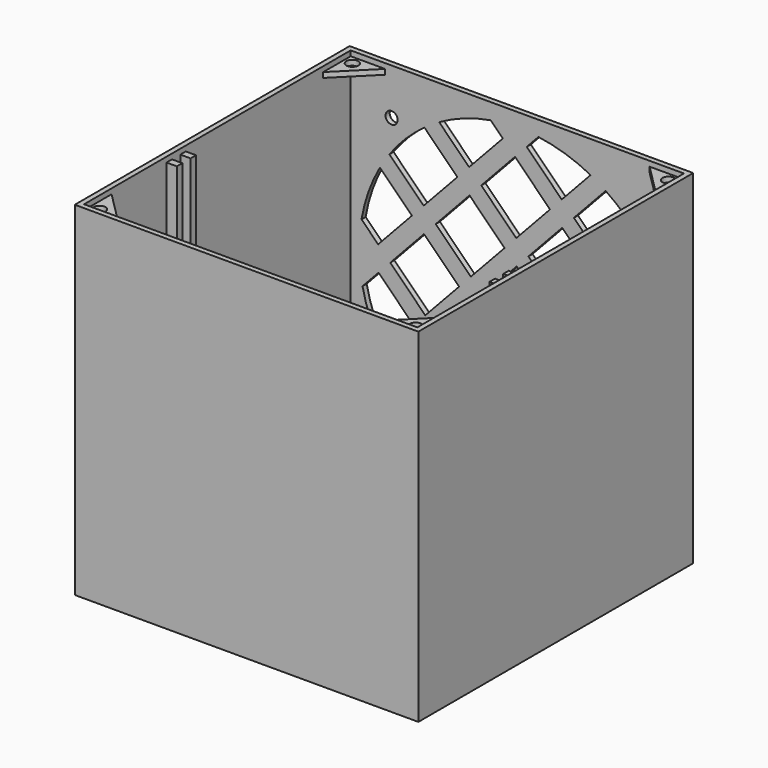
from build123d import *

# Parameters (mm, degrees)
F0_W      = 100
F0_H      = 100
F0_R      = 5
F0_W_2    = 3
F0_H_2    = 2
F1_DEPTH  = 1.5
F2_W      = 100
F2_H      = 100
F3_DEPTH  = 98.5
F2_W_2    = 3
F2_H_2    = 2
F4_DEPTH  = 97
F5_R      = 1.75
F6_DEPTH  = 1.5
F7_R      = 1.75
F8_DEPTH  = 3
F8_FACE_R = 1.75
F9_DEPTH  = 1.5
F2_R      = 3.5
F2_R_2    = 1.75
F10_DEPTH = 7


with BuildPart() as f1:
    # F0 (on Top) → F1 (new body)
    with BuildSketch(Plane.XY):
        with Locations((50, 50)):
            Rectangle(F0_W, F0_H)
        Polygon((98.5, 1.5), (1.5, 1.5), (1.5, 31.5), (1.5, 33.5), (1.5, 36.5), (1.5, 38.5), (1.5, 98.5), (98.5, 98.5), (98.5, 38.5), (98.5, 36.5), (98.5, 33.5), (98.5, 31.5), align=None, mode=Mode.SUBTRACT)
        Polygon((1.5, 31.5), (1.5, 1.5), (98.5, 1.5), (98.5, 31.5), (95.5, 31.5), (95.5, 33.5), (98.5, 33.5), (98.5, 36.5), (95.5, 36.5), (95.5, 38.5), (98.5, 38.5), (98.5, 98.5), (1.5, 98.5), (1.5, 38.5), (4.5, 38.5), (4.5, 36.5), (1.5, 36.5), (1.5, 33.5), (4.5, 33.5), (4.5, 31.5), align=None)
        with Locations((20.9, 53.5)):
            Circle(F0_R, mode=Mode.SUBTRACT)
        with Locations((40.3, 53.5)):
            Circle(F0_R, mode=Mode.SUBTRACT)
        with Locations((20.9, 78.5)):
            Circle(F0_R, mode=Mode.SUBTRACT)
        with Locations((59.7, 53.5)):
            Circle(F0_R, mode=Mode.SUBTRACT)
        with Locations((79.1, 53.5)):
            Circle(F0_R, mode=Mode.SUBTRACT)
        with Locations((79.1, 78.5)):
            Circle(F0_R, mode=Mode.SUBTRACT)
        with Locations((3, 37.5)):
            Rectangle(F0_W_2, F0_H_2)
        with Locations((3, 32.5)):
            Rectangle(F0_W_2, F0_H_2)
        with Locations((97, 37.5)):
            Rectangle(F0_W_2, F0_H_2)
        with Locations((97, 32.5)):
            Rectangle(F0_W_2, F0_H_2)
    extrude(amount=F1_DEPTH)

    # F2 (on face) → F3 (join)
    with BuildSketch(Plane.XY.offset(1.5)):
        with Locations((50, 50)):
            Rectangle(F2_W, F2_H)
        Polygon((98.5, 1.5), (1.5, 1.5), (1.5, 31.5), (1.5, 33.5), (1.5, 36.5), (1.5, 38.5), (1.5, 98.5), (98.5, 98.5), (98.5, 38.5), (98.5, 36.5), (98.5, 33.5), (98.5, 31.5), align=None, mode=Mode.SUBTRACT)
    extrude(amount=F3_DEPTH)

    # F2 (on face) → F4 (join)
    with BuildSketch(Plane.XY.offset(1.5)):
        with Locations((50, 50)):
            Rectangle(F2_W, F2_H)
        Polygon((98.5, 1.5), (1.5, 1.5), (1.5, 31.5), (1.5, 33.5), (1.5, 36.5), (1.5, 38.5), (1.5, 98.5), (98.5, 98.5), (98.5, 38.5), (98.5, 36.5), (98.5, 33.5), (98.5, 31.5), align=None, mode=Mode.SUBTRACT)
        with Locations((3, 37.5)):
            Rectangle(F2_W_2, F2_H_2)
        with Locations((3, 32.5)):
            Rectangle(F2_W_2, F2_H_2)
        with Locations((97, 37.5)):
            Rectangle(F2_W_2, F2_H_2)
        with Locations((97, 32.5)):
            Rectangle(F2_W_2, F2_H_2)
    extrude(amount=F4_DEPTH)

    # F5 (on face) → F6 (cut)
    with BuildSketch(Plane(origin=(0, 100, 0), x_dir=(-1, 0, 0), z_dir=(0, 1, 0))):
        with BuildLine():
            Line((-9.4901794257, 52.8917398152), (-4.6538158404, 57.7281034004))
            ThreePointArc((-4.6538158404, 57.7281034004), (-6.6777348094, 65.4654886362), (-10.0112182568, 72.7353762822))
            Line((-10.0112182568, 72.7353762822), (-19.3166099549, 63.4299845841))
            Line((-19.3166099549, 63.4299845841), (-9.4901794257, 52.8917398152))
        make_face()
        with BuildLine():
            ThreePointArc((-10.8298170716, 25.8816093125), (-7.24441602, 33.0306146685), (-4.9514495581, 40.6925780646))
            Line((-4.9514495581, 40.6925780646), (-9.615917377, 45.694934052))
            Line((-9.615917377, 45.694934052), (-19.8044732059, 35.5063782232))
            Line((-19.8044732059, 35.5063782232), (-10.8298170716, 25.8816093125))
        make_face()
        with BuildLine():
            Line((-22.7285649998, 67.0890973511), (-12.7828292456, 77.0348331054))
            ThreePointArc((-12.7828292456, 77.0348331054), (-17.4730880654, 82.5269119346), (-22.9651668946, 87.2171707544))
            Line((-22.9651668946, 87.2171707544), (-32.554995529, 77.62734212))
            Line((-32.554995529, 77.62734212), (-22.7285649998, 67.0890973511))
        make_face()
        Polygon((-23.2164282507, 39.1654909901), (-13.0278724219, 49.354046819), (-22.8543029511, 59.892291588), (-33.04285878, 49.7037357591), align=None)
        with BuildLine():
            ThreePointArc((-24.2817385198, 11.8611611814), (-18.6291712168, 16.3567079278), (-13.7499253493, 21.6815945396))
            Line((-13.7499253493, 21.6815945396), (-23.342166202, 31.968685227))
            Line((-23.342166202, 31.968685227), (-33.5307220309, 21.7801293981))
            Line((-33.5307220309, 21.7801293981), (-24.2817385198, 11.8611611814))
        make_face()
        with BuildLine():
            Line((-35.9669505739, 81.286454887), (-27.2646237178, 89.9887817432))
            ThreePointArc((-27.2646237178, 89.9887817432), (-34.5345113638, 93.3222651906), (-42.2718965996, 95.3461841596))
            Line((-42.2718965996, 95.3461841596), (-45.7933811031, 91.824699656))
            Line((-45.7933811031, 91.824699656), (-35.9669505739, 81.286454887))
        make_face()
        Polygon((-36.4548138248, 53.3628485261), (-26.266257996, 63.551404355), (-36.0926885252, 74.0896491239), (-46.281244354, 63.901093295), align=None)
        Polygon((-36.9426770757, 25.4392421651), (-26.7541212469, 35.627797994), (-36.5805517761, 46.166042763), (-46.769107605, 35.9774869341), align=None)
        with BuildLine():
            ThreePointArc((-43.8606482155, 4.4115326024), (-36.0572855508, 6.1639336415), (-28.6753893881, 9.2414305667))
            Line((-28.6753893881, 9.2414305667), (-37.068415027, 18.242436402))
            Line((-37.068415027, 18.242436402), (-47.2569708559, 8.0538805731))
            Line((-47.2569708559, 8.0538805731), (-43.8606482155, 4.4115326024))
        make_face()
        Polygon((-49.6931993989, 67.560206062), (-39.50464357, 77.7487618909), (-49.3310740993, 88.2870066599), (-59.5196299281, 78.098450831), align=None)
        Polygon((-50.1810626498, 39.6365997011), (-39.992506821, 49.82515553), (-49.8189373502, 60.3634002989), (-60.007493179, 50.17484447), align=None)
        Polygon((-50.6689259007, 11.7129933401), (-40.4803700719, 21.901549169), (-50.3068006011, 32.439793938), (-60.49535643, 22.2512381091), align=None)
        with BuildLine():
            Line((-52.7430291441, 91.9461194269), (-56.1393517845, 95.5884673976))
            ThreePointArc((-56.1393517845, 95.5884673976), (-63.9427144492, 93.8360663585), (-71.3246106119, 90.7585694333))
            Line((-71.3246106119, 90.7585694333), (-62.931584973, 81.757563598))
            Line((-62.931584973, 81.757563598), (-52.7430291441, 91.9461194269))
        make_face()
        Polygon((-63.4194482239, 53.833957237), (-53.230892395, 64.0225130659), (-63.0573229243, 74.5607578349), (-73.2458787531, 64.372202006), align=None)
        Polygon((-63.9073114748, 25.9103508761), (-53.718755646, 36.098906705), (-63.5451861752, 46.6371514739), (-73.733742004, 36.448595645), align=None)
        with BuildLine():
            Line((-57.7281034004, 4.6538158404), (-54.2066188969, 8.175300344))
            Line((-54.2066188969, 8.175300344), (-64.0330494261, 18.713545113))
            Line((-64.0330494261, 18.713545113), (-72.7353762822, 10.0112182568))
            ThreePointArc((-72.7353762822, 10.0112182568), (-65.4654886362, 6.6777348094), (-57.7281034004, 4.6538158404))
        make_face()
        with BuildLine():
            Line((-66.4692779691, 78.2198706019), (-75.7182614802, 88.1388388186))
            ThreePointArc((-75.7182614802, 88.1388388186), (-81.3708287832, 83.6432920722), (-86.2500746507, 78.3184054604))
            Line((-86.2500746507, 78.3184054604), (-76.657833798, 68.031314773))
            Line((-76.657833798, 68.031314773), (-66.4692779691, 78.2198706019))
        make_face()
        Polygon((-77.1456970489, 40.107708412), (-66.95714122, 50.2962642409), (-76.7835717493, 60.8345090099), (-86.9721275781, 50.645953181), align=None)
        with BuildLine():
            Line((-77.0348331054, 12.7828292456), (-67.445004471, 22.37265788))
            Line((-67.445004471, 22.37265788), (-77.2714350002, 32.9109026489))
            Line((-77.2714350002, 32.9109026489), (-87.2171707544, 22.9651668946))
            ThreePointArc((-87.2171707544, 22.9651668946), (-82.5269119346, 17.4730880654), (-77.0348331054, 12.7828292456))
        make_face()
        with BuildLine():
            Line((-80.1955267941, 64.4936217768), (-89.1701829284, 74.1183906875))
            ThreePointArc((-89.1701829284, 74.1183906875), (-92.75558398, 66.9693853315), (-95.0485504419, 59.3074219354))
            Line((-95.0485504419, 59.3074219354), (-90.384082623, 54.305065948))
            Line((-90.384082623, 54.305065948), (-80.1955267941, 64.4936217768))
        make_face()
        with BuildLine():
            Line((-89.9887817432, 27.2646237178), (-80.6833900451, 36.5700154159))
            Line((-80.6833900451, 36.5700154159), (-90.5098205743, 47.1082601848))
            Line((-90.5098205743, 47.1082601848), (-95.3461841596, 42.2718965996))
            ThreePointArc((-95.3461841596, 42.2718965996), (-93.3222651906, 34.5345113638), (-89.9887817432, 27.2646237178))
        make_face()
        with Locations((-13.4072240736, 86.5927759264)):
            Circle(F5_R)
        with Locations((-86.5927759264, 86.5927759264)):
            Circle(F5_R)
        with Locations((-86.5927759264, 13.4072240736)):
            Circle(F5_R)
        with Locations((-13.4072240736, 13.4072240736)):
            Circle(F5_R)
    extrude(amount=-F6_DEPTH, mode=Mode.SUBTRACT)

    # F2 (on face) → F10 (join)
    with BuildSketch(Plane.XY.offset(1.5)):
        with Locations((8.5, 78.5)):
            Circle(F2_R)
        with Locations((8.5, 78.5)):
            Circle(F2_R_2, mode=Mode.SUBTRACT)
        with Locations((91.5, 78.5)):
            Circle(F2_R)
        with Locations((91.5, 78.5)):
            Circle(F2_R_2, mode=Mode.SUBTRACT)
        with Locations((91.5, 53.5)):
            Circle(F2_R)
        with Locations((91.5, 53.5)):
            Circle(F2_R_2, mode=Mode.SUBTRACT)
        with Locations((8.5, 53.5)):
            Circle(F2_R)
        with Locations((8.5, 53.5)):
            Circle(F2_R_2, mode=Mode.SUBTRACT)
    extrude(amount=F10_DEPTH)


with BuildPart() as f8:
    # F7 (on face) → F8 (new body)
    with BuildSketch(Plane.XY.offset(100)):
        Polygon((11.5, 98.5), (1.5, 98.5), (1.5, 88.5), align=None)
        with Locations((4, 96)):
            Circle(F7_R, mode=Mode.SUBTRACT)
    extrude(amount=-F8_DEPTH)


with BuildPart() as f8b:
    # F7 (on face) → F8, piece 2 (new body)
    with BuildSketch(Plane.XY.offset(100)):
        Polygon((98.5, 98.5), (88.5, 98.5), (98.5, 88.5), align=None)
        with Locations((96, 96)):
            Circle(F7_R, mode=Mode.SUBTRACT)
    extrude(amount=-F8_DEPTH)


with BuildPart() as f8c:
    # F7 (on face) → F8, piece 3 (new body)
    with BuildSketch(Plane.XY.offset(100)):
        Polygon((98.5, 1.5), (98.5, 11.5), (88.5, 1.5), align=None)
        with Locations((96, 4)):
            Circle(F7_R, mode=Mode.SUBTRACT)
    extrude(amount=-F8_DEPTH)


with BuildPart() as f8d:
    # F7 (on face) → F8, piece 4 (new body)
    with BuildSketch(Plane.XY.offset(100)):
        Polygon((11.5, 1.5), (1.5, 11.5), (1.5, 1.5), align=None)
        with Locations((4, 4)):
            Circle(F7_R, mode=Mode.SUBTRACT)
    extrude(amount=-F8_DEPTH)


with BuildPart() as f9_tool:
    # F8_face (on face) → F9 (new body)
    with BuildSketch(Plane(origin=(5.0318927719, 94.9681072281, 100), x_dir=(1, 0, 0), z_dir=(0, 0, 1))):
        Polygon((6.4681072281, 3.5318927719), (-3.5318927719, 3.5318927719), (-3.5318927719, -6.4681072281), align=None)
        with Locations((-1.0318927719, 1.0318927719)):
            Circle(F8_FACE_R, mode=Mode.SUBTRACT)
        Polygon((93.4681072281, 3.5318927719), (83.4681072281, 3.5318927719), (93.4681072281, -6.4681072281), align=None)
        with Locations((90.9681072281, 1.0318927719)):
            Circle(F8_FACE_R, mode=Mode.SUBTRACT)
        Polygon((93.4681072281, -93.4681072281), (93.4681072281, -83.4681072281), (83.4681072281, -93.4681072281), align=None)
        with Locations((90.9681072281, -90.9681072281)):
            Circle(F8_FACE_R, mode=Mode.SUBTRACT)
        Polygon((6.4681072281, -93.4681072281), (-3.5318927719, -83.4681072281), (-3.5318927719, -93.4681072281), align=None)
        with Locations((-1.0318927719, -90.9681072281)):
            Circle(F8_FACE_R, mode=Mode.SUBTRACT)
    extrude(amount=-F9_DEPTH)


with BuildPart() as f8_1:
    add(f8.part)

    # F9: cut by f9_tool
    add(f9_tool.part, mode=Mode.SUBTRACT)


with BuildPart() as f8b_1:
    add(f8b.part)

    # F9: cut by f9_tool
    add(f9_tool.part, mode=Mode.SUBTRACT)


with BuildPart() as f8c_1:
    add(f8c.part)

    # F9: cut by f9_tool
    add(f9_tool.part, mode=Mode.SUBTRACT)


with BuildPart() as f8d_1:
    add(f8d.part)

    # F9: cut by f9_tool
    add(f9_tool.part, mode=Mode.SUBTRACT)


solid = Compound([f1.part, f8_1.part, f8b_1.part, f8c_1.part, f8d_1.part])
